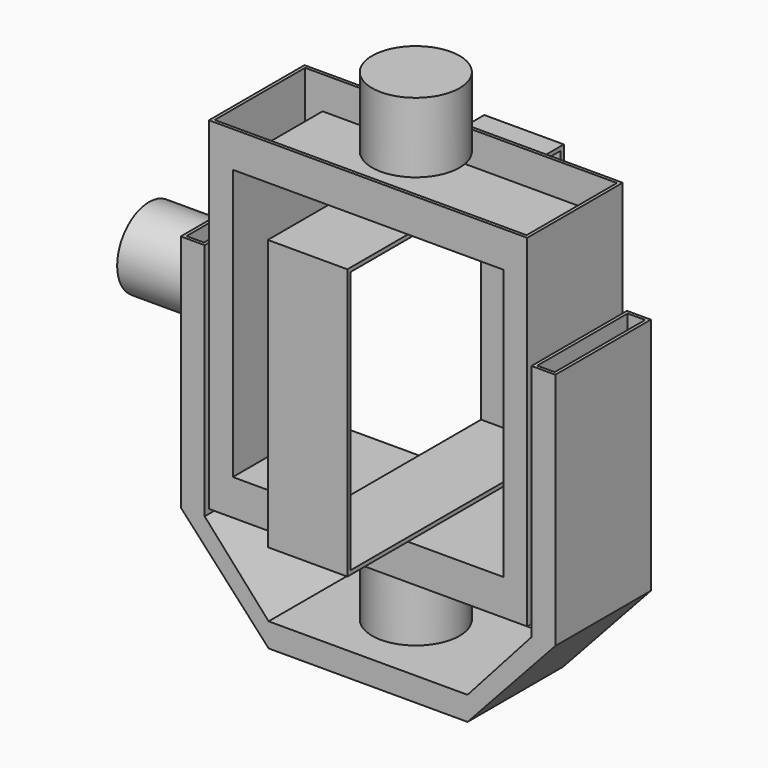
from build123d import *

# Parameters (mm, degrees)
F0_W      = 340
F0_H      = 340
F0_W_2    = 330
F0_H_2    = 330
F1_DEPTH  = 50
F2_W      = 400
F2_H      = 430
F2_W_2    = 340
F2_H_2    = 340
F3_DEPTH  = 75
F4_W      = 30
F4_H      = 300
F4_W_2    = 250
F4_H_2    = 30
F5_DEPTH  = 75
F6_T      = -4
F8_T      = -4
F7_R      = 50
F9_DEPTH  = 100
F10_R     = 55
F11_DEPTH = 88


# Not quite as in the source:
# - a pattern or mirror of a feature is missing from the dataset's text; its kind, count and spacing are read off the source's solid


with BuildPart() as f1:
    # F0 (on Right) → F1 (new body, symmetric)
    with BuildSketch(Plane.YZ):
        Rectangle(F0_W, F0_H)
        Rectangle(F0_W_2, F0_H_2, mode=Mode.SUBTRACT)
    extrude(amount=F1_DEPTH, both=True)


with BuildPart() as f3:
    # F2 (on Front) → F3 (new body, symmetric)
    with BuildSketch(Plane.XZ):
        Rectangle(F2_W, F2_H)
        Rectangle(F2_W_2, F2_H_2, mode=Mode.SUBTRACT)
    extrude(amount=F3_DEPTH, both=True)

    # F8
    f8_openings = [f3.faces().sort_by_distance(p)[0] for p in [
        (0, 0, 215),
    ]]
    offset(amount=F8_T, openings=f8_openings, kind=Kind.INTERSECTION)

    # F10 (on face) → F11 (join)
    with BuildSketch(Plane(origin=(0, 0, -215), x_dir=(1, 0, 0), z_dir=(0, 0, -1))):
        Circle(F10_R)
    f11 = extrude(amount=F11_DEPTH)

    # F11_copies: F11 across plane
    add(f11.mirror(Plane.XY))


with BuildPart() as f5:
    # F4 (on Front) → F5 (new body, symmetric)
    with BuildSketch(Plane.XZ):
        with Locations((-220.3749617156, -75)):
            Rectangle(F4_W, F4_H)
        Polygon((-205.3749617156, -225), (-235.3749617156, -225), (-125, -345), (-125, -315), align=None)
        with Locations((0, -330)):
            Rectangle(F4_W_2, F4_H_2)
        Polygon((125, -315), (125, -345), (235.3749617156, -225), (235.3749617156, 75), (205.3749617156, 75), (205.3749617156, -225), align=None)
    extrude(amount=F5_DEPTH, both=True)

    # F6
    f6_openings = [f5.faces().sort_by_distance(p)[0] for p in [
        (-220.374962, 0, 75),
        (220.374962, 0, 75),
    ]]
    offset(amount=F6_T, openings=f6_openings, kind=Kind.INTERSECTION)

    # F7 (on face) → F9 (join)
    with BuildSketch(Plane(origin=(-235.3749617156, 0, 0), x_dir=(0, -1, 0), z_dir=(-1, 0, 0))):
        Circle(F7_R)
    extrude(amount=F9_DEPTH)


solid = Compound([f1.part, f3.part, f5.part])
